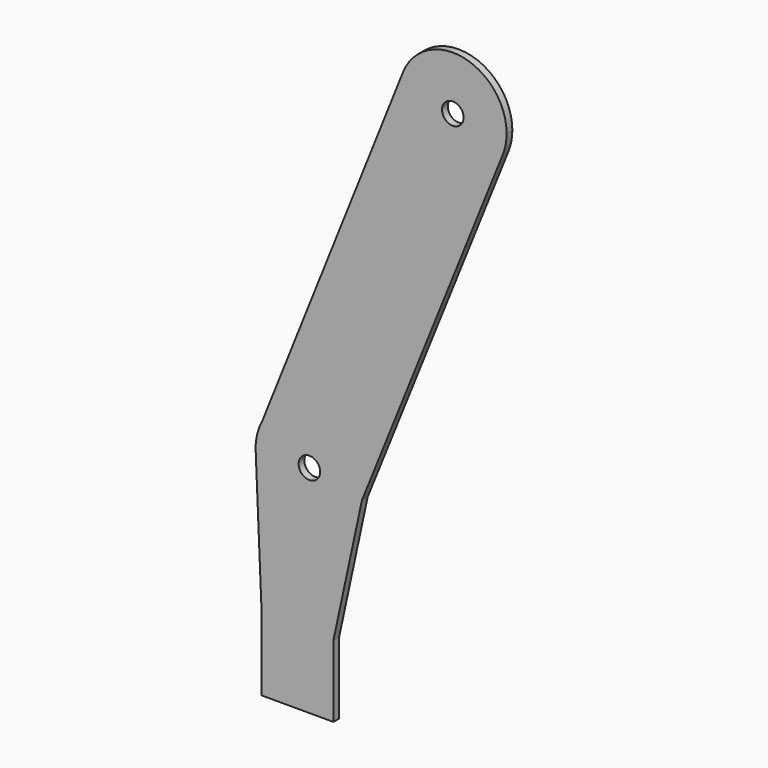
from build123d import *

# Parameters (mm, degrees)
F0_W     = 100
F0_H     = 100
F0_R     = 15
F1_DEPTH = 10


# Not quite as in the source:
# - a feature names something its author has since deleted; it is built from what else it names


with BuildPart() as f1:
    # F0 (on Front) → F1 (new body)
    with BuildSketch(Plane.XZ):
        with Locations((-366.5186442992, -742.7781961888)):
            Rectangle(F0_W, F0_H)
        with BuildLine():
            Line((-424.891556994, -494.917224318), (-416.5186442992, -692.7781961888))
            Line((-416.5186442992, -692.7781961888), (-316.5186442992, -692.7781961888))
            Line((-316.5186442992, -692.7781961888), (-276.6384194866, -507.5307060219))
            ThreePointArc((-276.6384194866, -507.5307060219), (-356.3167020216, -566.4762885136), (-424.891556994, -494.917224318))
        make_face()
        with BuildLine():
            ThreePointArc((-415.8601836979, -455.9414735734), (-423.022745475, -474.8160209943), (-424.891556994, -494.917224318))
            ThreePointArc((-424.891556994, -494.917224318), (-356.3167020216, -566.4762885136), (-276.6384194866, -507.5307060219))
            ThreePointArc((-276.6384194866, -507.5307060219), (-275.3797520239, -499.6830567418), (-274.9586197372, -491.7462758703))
            ThreePointArc((-274.9586197372, -491.7462758703), (-331.4872540196, -419.0564646962), (-415.8601836979, -455.9414735734))
        make_face()
        with Locations((-349.9586197372, -491.7462758703)):
            Circle(F0_R, mode=Mode.SUBTRACT)
        with BuildLine():
            ThreePointArc((-274.9586197372, -491.7462758703), (-275.3797520239, -499.6830567418), (-276.6384194866, -507.5307060219))
            Line((-276.6384194866, -507.5307060219), (-80.3792470285, -19.7411127776))
            ThreePointArc((-80.3792470285, -19.7411127776), (-177.8494040627, -61.3674231584), (-219.6213859991, 36.0403935367))
            Line((-219.6213859991, 36.0403935367), (-415.8601836979, -455.9414735734))
            ThreePointArc((-415.8601836979, -455.9414735734), (-331.4872540196, -419.0564646962), (-274.9586197372, -491.7462758703))
        make_face()
        with BuildLine():
            ThreePointArc((-219.6213859991, 36.0403935367), (-177.8494040627, -61.3674231584), (-80.3792470285, -19.7411127776))
            ThreePointArc((-80.3792470285, -19.7411127776), (-76.3262459022, -6.0036782783), (-74.9586197372, 8.2537241297))
            ThreePointArc((-74.9586197372, 8.2537241297), (-135.8113138036, 81.9073305236), (-219.6213859991, 36.0403935367))
        make_face()
        with Locations((-149.9586197372, 8.2537241297)):
            Circle(F0_R, mode=Mode.SUBTRACT)
    extrude(amount=F1_DEPTH)


solid = f1.part
